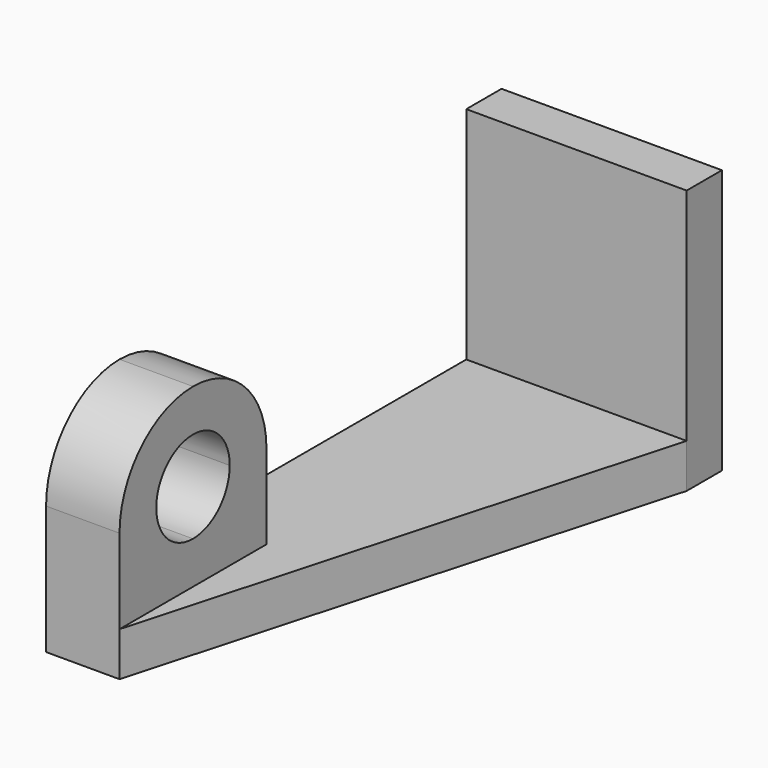
from build123d import *

# Parameters (mm, degrees)
F1_DEPTH  = 30.48
F3_DEPTH  = 30.48
F5_DEPTH  = 30.48
F6_W      = 152.4
F6_H      = 30.48
F7_DEPTH  = 152.4
F8_W      = 50.8
F8_H      = 127
F9_DEPTH  = 121.92
F11_DEPTH = 475.742
F12_R     = 63.49999


# Not quite as in the source:
# - a fillet or chamfer is up to 0.001 mm smaller than in the source, because OpenCascade refuses the exact size


with BuildPart() as f1:
    # F0 (on Top) → F1 (new body)
    with BuildSketch(Plane.XY):
        Polygon((152.4, 0), (0, 0), (0, -393.7), (50.8, -393.7), align=None)
    extrude(amount=F1_DEPTH)

    # F2 (on face) → F3 (join)
    with BuildSketch(Plane.XY.offset(30.48)):
        Polygon((152.4, -30.48), (152.4, 0), (144.5341935484, -30.48), align=None)
    extrude(amount=-F3_DEPTH)

    # F4 (on face) → F5 (join)
    with BuildSketch(Plane.XY.offset(30.48)):
        Polygon((50.8, -393.7), (152.4, -30.48), (144.5341935484, -30.48), align=None)
    extrude(amount=-F5_DEPTH)

    # F6 (on face) → F7 (join)
    with BuildSketch(Plane.XY.offset(30.48)):
        with Locations((76.2, -15.24)):
            Rectangle(F6_W, F6_H)
    extrude(amount=F7_DEPTH)

    # F8 (on face) → F9 (join)
    with BuildSketch(Plane.XY.offset(30.48)):
        with Locations((25.4, -330.2)):
            Rectangle(F8_W, F8_H)
    extrude(amount=F9_DEPTH)

    # F10 (on face) → F11 (cut)
    with BuildSketch(Plane.YZ.offset(50.8)):
        with BuildLine():
            Line((-330.2, 91.44), (-330.2, 123.19))
            ThreePointArc((-330.2, 123.19), (-352.6506403027, 113.8906403027), (-361.95, 91.44))
            Line((-361.95, 91.44), (-330.2, 91.44))
        make_face()
        with BuildLine():
            ThreePointArc((-298.45, 91.44), (-307.7493596973, 113.8906403027), (-330.2, 123.19))
            Line((-330.2, 123.19), (-330.2, 91.44))
            Line((-330.2, 91.44), (-298.45, 91.44))
        make_face()
        with BuildLine():
            Line((-330.2, 59.69), (-330.2, 91.44))
            Line((-330.2, 91.44), (-361.95, 91.44))
            ThreePointArc((-361.95, 91.44), (-352.6506403027, 68.9893596973), (-330.2, 59.69))
        make_face()
        with BuildLine():
            ThreePointArc((-330.2, 59.69), (-307.7493596973, 68.9893596973), (-298.45, 91.44))
            Line((-298.45, 91.44), (-330.2, 91.44))
            Line((-330.2, 91.44), (-330.2, 59.69))
        make_face()
    extrude(amount=-F11_DEPTH, mode=Mode.SUBTRACT)

    # F12 (radius 63.5 in the source; OpenCascade refuses exactly that, so slightly less here)
    f12_edges = [f1.edges().sort_by_distance(p)[0] for p in [
        (25.4, -393.7, 152.4),
        (25.4, -266.7, 152.4),
    ]]
    fillet(f12_edges, radius=F12_R)


solid = f1.part
